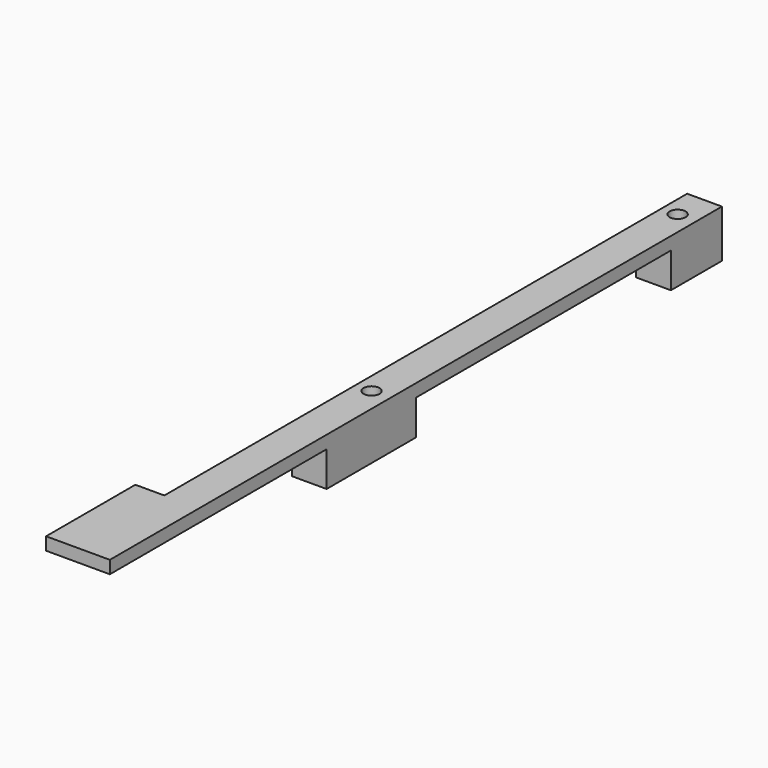
from build123d import *

# Parameters (mm, degrees)
F1_DEPTH = 304.8
F3_D     = 12.7
F4_W     = 27.686
F4_H     = 215.9
F4_H_2   = 254
F5_DEPTH = 27.94
F6_W     = 23.114
F6_H     = 520.7
F7_DEPTH = 10.161


# Not quite as in the source:
# - a length typed as a fraction of an inch, garbled in the dataset ("3 / 203.2 mm" for 3/8 in), is restored


with BuildPart() as f1:
    # F0 (on Front) → F1 (new body, symmetric)
    with BuildSketch(Plane.XZ):
        Polygon((0, 27.94), (0, 0), (27.686, 0), (27.686, 38.1), (-23.114, 38.1), (-23.114, 27.94), align=None)
    extrude(amount=F1_DEPTH, both=True)

    # F3 (through all)
    with Locations(Plane(origin=(0, 0, 0), x_dir=(1, 0, 0), z_dir=(0, 0, -1))):
        with Locations((12.7, 25.4), (12.7, -279.4)):
            Hole(F3_D / 2)

    # F4 (on face) → F5 (cut, through all)
    with BuildSketch(Plane(origin=(0, 0, 0), x_dir=(1, 0, 0), z_dir=(0, 0, -1))):
        with Locations((13.843, 196.85)):
            Rectangle(F4_W, F4_H)
        with Locations((13.843, -127)):
            Rectangle(F4_W, F4_H_2)
    extrude(amount=-F5_DEPTH, mode=Mode.SUBTRACT)

    # F6 (on face) → F7 (cut, through all)
    with BuildSketch(Plane(origin=(0, 0, 27.94), x_dir=(1, 0, 0), z_dir=(0, 0, -1))):
        with Locations((-11.557, -44.45)):
            Rectangle(F6_W, F6_H)
    extrude(amount=-F7_DEPTH, mode=Mode.SUBTRACT)


solid = f1.part
